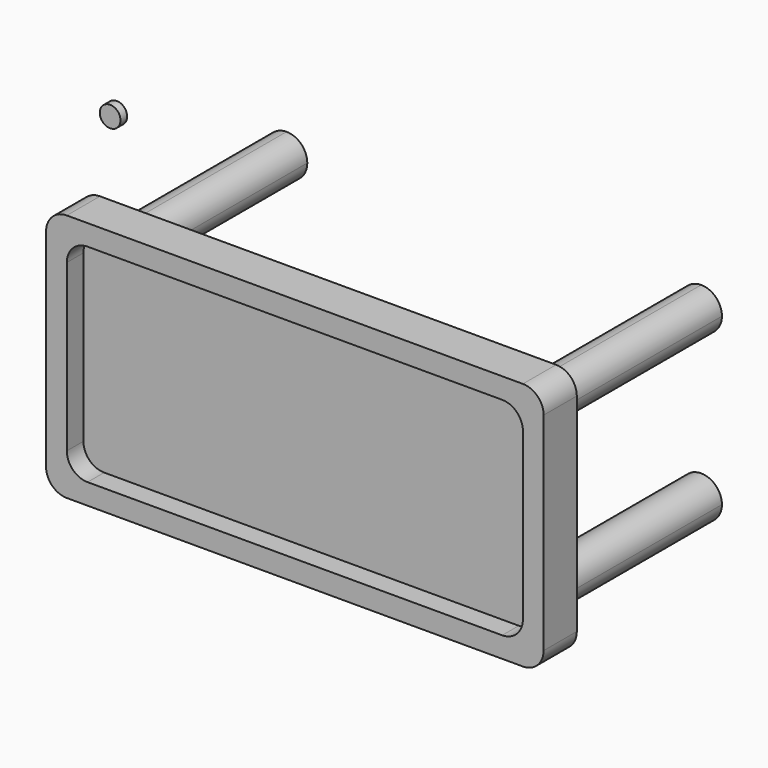
from build123d import *

# Parameters (mm, degrees)
F1_DEPTH = 12.7
F2_DEPTH = 63.5
F3_DEPTH = 6.35
F4_R     = 3.175
F5_DEPTH = 2.54


with BuildPart() as f1:
    # F0 (on Front) → F1 (new body)
    with BuildSketch(Plane.XZ):
        with BuildLine():
            Line((69.85, 38.1), (-69.85, 38.1))
            ThreePointArc((-69.85, 38.1), (-74.3401280605, 36.2401280605), (-76.2, 31.75))
            Line((-76.2, 31.75), (-76.2, -31.75))
            ThreePointArc((-76.2, -31.75), (-74.3401280605, -36.2401280605), (-69.85, -38.1))
            Line((-69.85, -38.1), (69.85, -38.1))
            ThreePointArc((69.85, -38.1), (74.3401280605, -36.2401280605), (76.2, -31.75))
            Line((76.2, -31.75), (76.2, 31.75))
            ThreePointArc((76.2, 31.75), (74.3401280605, 36.2401280605), (69.85, 38.1))
        make_face()
        with BuildLine():
            ThreePointArc((-69.85, 25.4), (-67.9901280605, 29.8901280605), (-63.5, 31.75))
            Line((-63.5, 31.75), (63.5, 31.75))
            ThreePointArc((63.5, 31.75), (67.9901280605, 29.8901280605), (69.85, 25.4))
            Line((69.85, 25.4), (69.85, -25.4))
            ThreePointArc((69.85, -25.4), (67.9901280605, -29.8901280605), (63.5, -31.75))
            Line((63.5, -31.75), (-63.5, -31.75))
            ThreePointArc((-63.5, -31.75), (-67.9901280605, -29.8901280605), (-69.85, -25.4))
            Line((-69.85, -25.4), (-69.85, 25.4))
        make_face(mode=Mode.SUBTRACT)
    extrude(amount=F1_DEPTH)

    # F0 (on Front) → F3 (join)
    with BuildSketch(Plane.XZ):
        with BuildLine():
            Line((63.5, 31.75), (-63.5, 31.75))
            ThreePointArc((-63.5, 31.75), (-59.0098719395, 29.8901280605), (-57.15, 25.4))
            ThreePointArc((-57.15, 25.4), (-63.5, 19.05), (-69.85, 25.4))
            Line((-69.85, 25.4), (-69.85, -25.4))
            ThreePointArc((-69.85, -25.4), (-63.5, -19.05), (-57.15, -25.4))
            ThreePointArc((-57.15, -25.4), (-59.0098719395, -29.8901280605), (-63.5, -31.75))
            Line((-63.5, -31.75), (63.5, -31.75))
            ThreePointArc((63.5, -31.75), (59.0098719395, -20.9098719395), (69.85, -25.4))
            Line((69.85, -25.4), (69.85, 25.4))
            ThreePointArc((69.85, 25.4), (59.0098719395, 20.9098719395), (63.5, 31.75))
        make_face()
        with BuildLine():
            ThreePointArc((-57.15, 25.4), (-59.0098719395, 29.8901280605), (-63.5, 31.75))
            ThreePointArc((-63.5, 31.75), (-67.9901280605, 29.8901280605), (-69.85, 25.4))
            ThreePointArc((-69.85, 25.4), (-63.5, 19.05), (-57.15, 25.4))
        make_face()
        with BuildLine():
            ThreePointArc((69.85, 25.4), (67.9901280605, 29.8901280605), (63.5, 31.75))
            ThreePointArc((63.5, 31.75), (59.0098719395, 20.9098719395), (69.85, 25.4))
        make_face()
        with BuildLine():
            ThreePointArc((63.5, -31.75), (67.9901280605, -29.8901280605), (69.85, -25.4))
            ThreePointArc((69.85, -25.4), (59.0098719395, -20.9098719395), (63.5, -31.75))
        make_face()
        with BuildLine():
            ThreePointArc((-57.15, -25.4), (-63.5, -19.05), (-69.85, -25.4))
            ThreePointArc((-69.85, -25.4), (-67.9901280605, -29.8901280605), (-63.5, -31.75))
            ThreePointArc((-63.5, -31.75), (-59.0098719395, -29.8901280605), (-57.15, -25.4))
        make_face()
    extrude(amount=F3_DEPTH)


with BuildPart() as f2:
    # F0 (on Front) → F2 (new body)
    with BuildSketch(Plane.XZ):
        with BuildLine():
            ThreePointArc((-57.15, 25.4), (-59.0098719395, 29.8901280605), (-63.5, 31.75))
            ThreePointArc((-63.5, 31.75), (-67.9901280605, 29.8901280605), (-69.85, 25.4))
            ThreePointArc((-69.85, 25.4), (-63.5, 19.05), (-57.15, 25.4))
        make_face()
    extrude(amount=-F2_DEPTH)


with BuildPart() as f2b:
    # F0 (on Front) → F2, piece 2 (new body)
    with BuildSketch(Plane.XZ):
        with BuildLine():
            ThreePointArc((-57.15, -25.4), (-63.5, -19.05), (-69.85, -25.4))
            ThreePointArc((-69.85, -25.4), (-67.9901280605, -29.8901280605), (-63.5, -31.75))
            ThreePointArc((-63.5, -31.75), (-59.0098719395, -29.8901280605), (-57.15, -25.4))
        make_face()
    extrude(amount=-F2_DEPTH)


with BuildPart() as f2c:
    # F0 (on Front) → F2, piece 3 (new body)
    with BuildSketch(Plane.XZ):
        with BuildLine():
            ThreePointArc((63.5, -31.75), (67.9901280605, -29.8901280605), (69.85, -25.4))
            ThreePointArc((69.85, -25.4), (59.0098719395, -20.9098719395), (63.5, -31.75))
        make_face()
    extrude(amount=-F2_DEPTH)


with BuildPart() as f2d:
    # F0 (on Front) → F2, piece 4 (new body)
    with BuildSketch(Plane.XZ):
        with BuildLine():
            ThreePointArc((69.85, 25.4), (67.9901280605, 29.8901280605), (63.5, 31.75))
            ThreePointArc((63.5, 31.75), (59.0098719395, 20.9098719395), (69.85, 25.4))
        make_face()
    extrude(amount=-F2_DEPTH)


with BuildPart() as f5:
    # F4 (on Front) → F5 (new body)
    with BuildSketch(Plane.XZ):
        with Locations((-64.708545804, 62.3119361699)):
            Circle(F4_R)
    extrude(amount=F5_DEPTH)


solid = Compound([f1.part, f2.part, f2b.part, f2c.part, f2d.part, f5.part])
